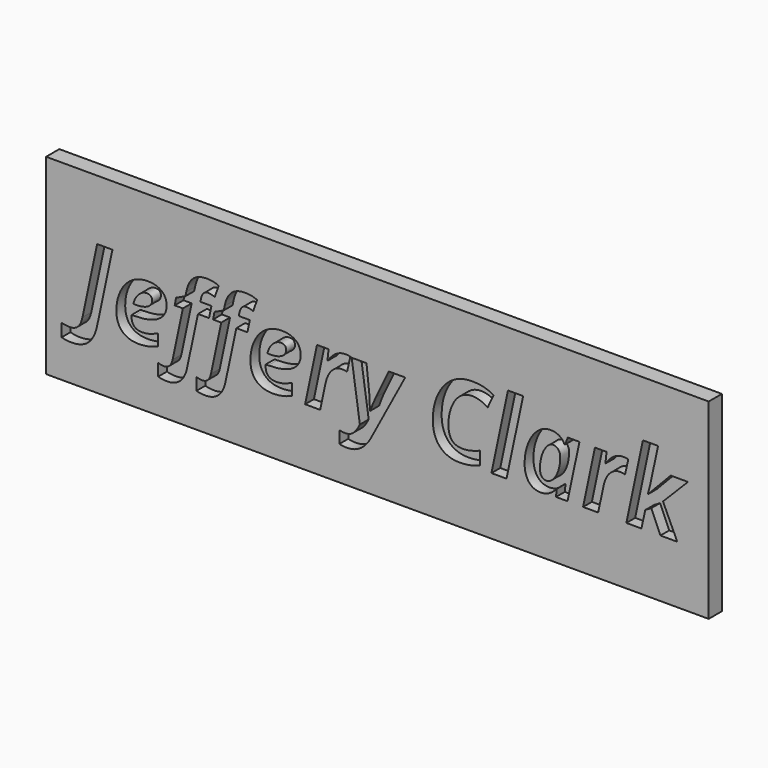
from build123d import *

# Parameters (mm, degrees)
F0_W         = 152.7060717344
F0_H         = 44.1052373499
F1_DEPTH     = 3.81
F2_TEXT_SIZE = 23.7025624503
F3_DEPTH     = 2.54


# Not quite as in the source:
# - Text() gives the source's letters only with a copy of the font that has no kerning and outlines rounded to 1/6400 em; it was checked with that copy


with BuildPart() as f1:
    # F0 (on Front) → F1 (new body)
    with BuildSketch(Plane.XZ):
        with Locations((-0.1108199358, 0.9973542765)):
            Rectangle(F0_W, F0_H)
    extrude(amount=F1_DEPTH)

    # F2 (on face) → F3 (cut)
    with BuildSketch(Plane.XZ.offset(3.81)):
        with Locations((-69.1499114037, -7.7572022565)):
            Text('Jeffery Clark', F2_TEXT_SIZE, font='Open Sans', font_style=FontStyle.BOLDITALIC, text_align=(TextAlign.LEFT, TextAlign.BOTTOM))
    extrude(amount=-F3_DEPTH, mode=Mode.SUBTRACT)


solid = f1.part
